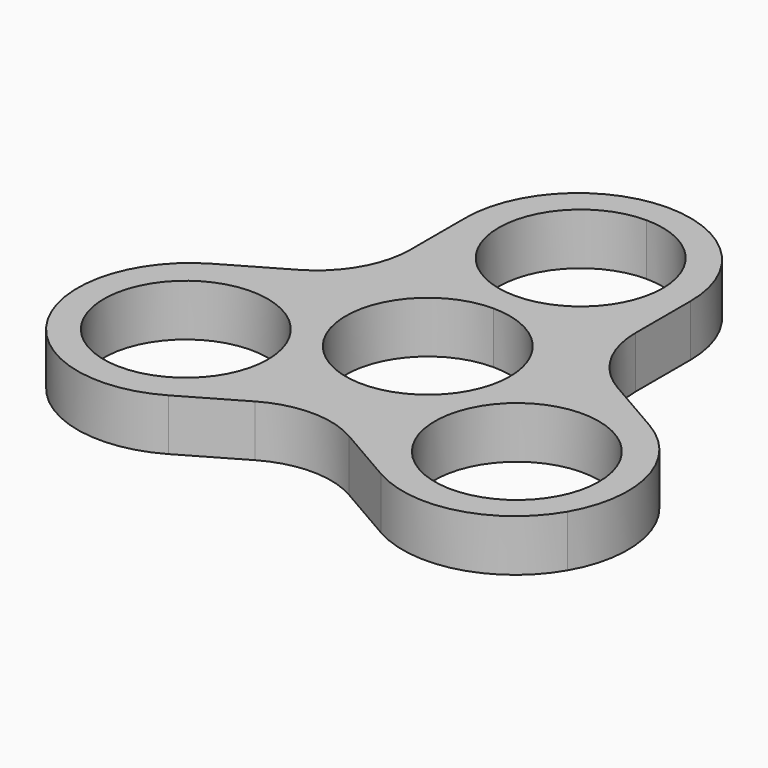
from build123d import *

# Parameters (mm, degrees)
F0_R     = 11.1
F1_DEPTH = 7
F2_R     = 15.23999
F3_R     = 12.7


# Not quite as in the source:
# - a fillet or chamfer is up to 0.001 mm smaller than in the source, because OpenCascade refuses the exact size


with BuildPart() as f1:
    # F0 (on Top) → F1 (new body)
    with BuildSketch(Plane.XY):
        Polygon((15.24, 40.64), (0, 40.64), (-15.24, 40.64), (-15.24, 8.7988181024), (-42.8152724098, -7.1217728463), (-27.5752724098, -33.5182271537), (0, -17.5976362049), (27.5752724098, -33.5182271537), (42.8152724098, -7.1217728463), (15.24, 8.7988181024), align=None)
        with Locations((-22.4040771959, -12.935)):
            Circle(F0_R, mode=Mode.SUBTRACT)
        with BuildLine():
            ThreePointArc((0, 11.1), (7.8488852712, 7.8488852712), (11.1, 0))
            ThreePointArc((11.1, 0), (-7.8488852712, -7.8488852712), (0, 11.1))
        make_face(mode=Mode.SUBTRACT)
        with Locations((22.4040771959, -12.935)):
            Circle(F0_R, mode=Mode.SUBTRACT)
        with BuildLine():
            ThreePointArc((11.1, 25.87), (7.8488852712, 18.0211147288), (0, 14.77))
            ThreePointArc((0, 14.77), (-11.1, 25.87), (0, 36.97))
            ThreePointArc((0, 36.97), (7.8488852712, 33.7188852712), (11.1, 25.87))
        make_face(mode=Mode.SUBTRACT)
    extrude(amount=F1_DEPTH)

    # F2 (radius 15.24 in the source; OpenCascade refuses exactly that, so slightly less here)
    f2_edges = [f1.edges().sort_by_distance(p)[0] for p in [
        (15.24, 40.64, 3.5),
        (-15.24, 40.64, 3.5),
        (-42.815272, -7.121773, 3.5),
        (-27.575272, -33.518227, 3.5),
        (42.815272, -7.121773, 3.5),
        (27.575272, -33.518227, 3.5),
    ]]
    fillet(f2_edges, radius=F2_R)

    # F3
    f3_edges = [f1.edges().sort_by_distance(p)[0] for p in [
        (15.24, 8.798818, 3.5),
        (0, -17.597636, 3.5),
        (-15.24, 8.798818, 3.5),
    ]]
    fillet(f3_edges, radius=F3_R)


solid = f1.part
